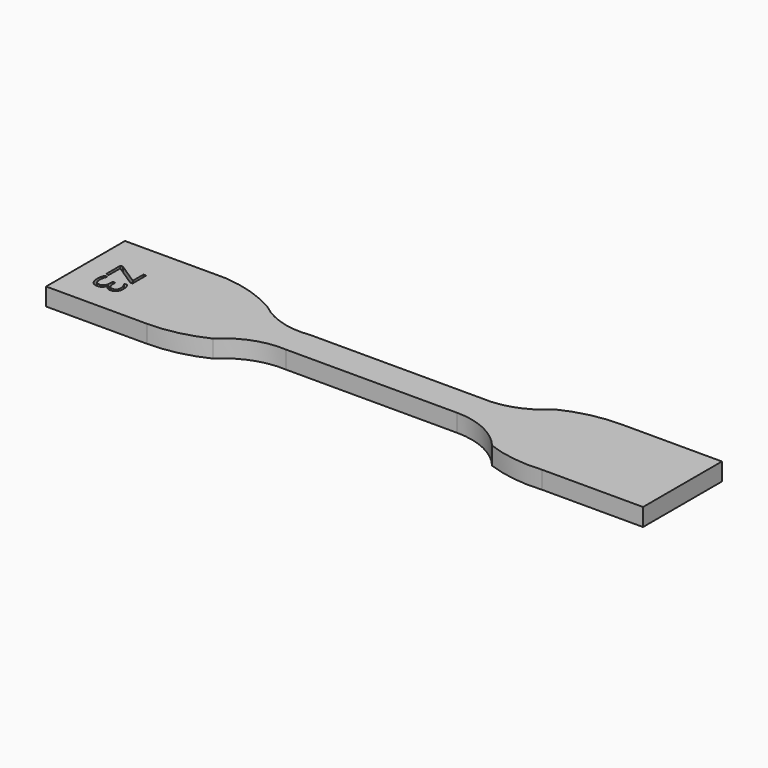
from build123d import *

# Parameters (mm, degrees)
F1_DEPTH     = 3.4
F2_TEXT_SIZE = 7.0564552314
F3_DEPTH     = 1


# Not quite as in the source:
# - Text() gives the source's letters only with a copy of the font that has no kerning and outlines rounded to 1/6400 em; it was checked with that copy


with BuildPart() as f1:
    # F0 (on Top) → F1 (new body)
    with BuildSketch(Plane.XY):
        with BuildLine():
            Line((-14.4320548165, 19.7811394548), (-33.8720548165, 19.7811394548))
            Line((-33.8720548165, 19.7811394548), (-33.8720548165, 0.7811394548))
            Line((-33.8720548165, 0.7811394548), (-14.4320548165, 0.7811394548))
            ThreePointArc((-14.4320548165, 0.7811394548), (-8.9053122052, 1.3996892086), (-3.6520548165, 3.2247301661))
            ThreePointArc((-3.6520548165, 3.2247301661), (1.3014698263, 6.4128780055), (7.1279451835, 7.2811394548))
            Line((7.1279451835, 7.2811394548), (40.1279451835, 7.2811394548))
            ThreePointArc((40.1279451835, 7.2811394548), (46.0837574042, 5.9511158081), (50.9079451835, 2.2137538538))
            ThreePointArc((50.9079451835, 2.2137538538), (56.2191047011, 0.9041953221), (61.6879451835, 0.7811394548))
            Line((61.6879451835, 0.7811394548), (81.1279451835, 0.7811394548))
            Line((81.1279451835, 0.7811394548), (81.1279451835, 19.7811394548))
            Line((81.1279451835, 19.7811394548), (61.6879451835, 19.7811394548))
            ThreePointArc((61.6879451835, 19.7811394548), (56.1612025723, 19.162589701), (50.9079451835, 17.3375487435))
            ThreePointArc((50.9079451835, 17.3375487435), (45.9544205407, 14.1494009041), (40.1279451835, 13.2811394548))
            Line((40.1279451835, 13.2811394548), (7.1279451835, 13.2811394548))
            ThreePointArc((7.1279451835, 13.2811394548), (1.4167452884, 13.6925537245), (-3.6520548165, 16.3560723447))
            ThreePointArc((-3.6520548165, 16.3560723447), (-8.8458057958, 18.686276846), (-14.4320548165, 19.7811394548))
        make_face()
    extrude(amount=F1_DEPTH)

    # F2 (on face) → F3 (cut)
    with BuildSketch(Plane.XY.offset(3.4)):
        with Locations(Location((-29.3720550835, 13.353464842), (0, 0, -90))):
            Text('Z3', F2_TEXT_SIZE, font='Open Sans', text_align=(TextAlign.LEFT, TextAlign.BOTTOM))
    extrude(amount=-F3_DEPTH, mode=Mode.SUBTRACT)


solid = f1.part
